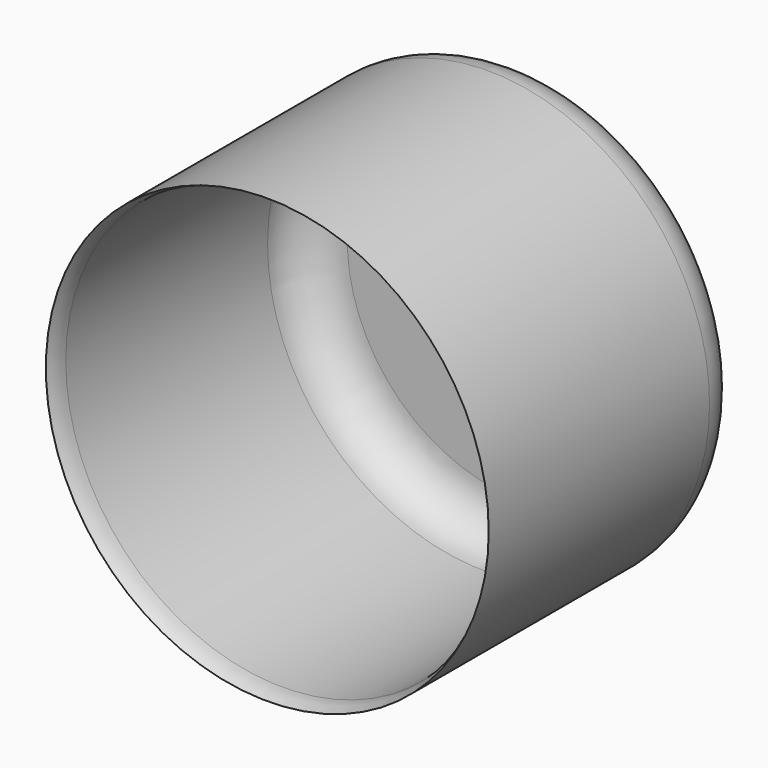
from build123d import *

# Parameters (mm, degrees)
F0_R     = 127
F1_DEPTH = 183.69425
F2_T     = -2.54


# Not quite as in the source:
# - a fillet or chamfer that OpenCascade refuses, or shapes differently, is made with other operations: its cross-section is extruded or revolved along the edge and cut away or added


with BuildPart() as f1:
    # F0 (on Front) → F1 (new body)
    with BuildSketch(Plane.XZ):
        Circle(F0_R)
    extrude(amount=F1_DEPTH)

    # F2
    f2_openings = [f1.faces().sort_by_distance(p)[0] for p in [
        (0, -183.69425, 0),
    ]]
    offset(amount=F2_T, openings=f2_openings)

    # F3: fillet of radius 25.4 on 3 edges, made by hand

    # F3_s1 → F3_t2 (revolve)
    with BuildSketch(Plane.XY):
        with BuildLine():
            ThreePointArc((124.46, -27.94), (117.0205122421, -9.9794877579), (99.06, -2.54))
            Line((99.06, -2.54), (124.46, -2.54))
            Line((124.46, -2.54), (124.46, -27.94))
        make_face()
    revolve(axis=Axis((0, -2.54, 0), (0, 1, 0)))

    # F3_s3 → F3_t4 (revolve, cut)
    with BuildSketch(Plane.XY):
        with BuildLine():
            ThreePointArc((127, -25.4), (119.5605122421, -7.4394877579), (101.6, 0))
            Line((101.6, 0), (127, 0))
            Line((127, 0), (127, -25.4))
        make_face()
    revolve(axis=Axis((0, 0, 0), (0, -1, 0)), mode=Mode.SUBTRACT)

    # F3_s5 → F3_t6 (revolve, cut)
    with BuildSketch(Plane.XY):
        with BuildLine():
            ThreePointArc((127, -183.69425), (125.1031423642, -178.3022593463), (124.46, -172.6226466834))
            Line((124.46, -172.6226466834), (124.46, -183.69425))
            Line((124.46, -183.69425), (127, -183.69425))
        make_face()
    revolve(axis=Axis((0, -183.69425, 0), (0, -1, 0)), mode=Mode.SUBTRACT)


solid = f1.part
